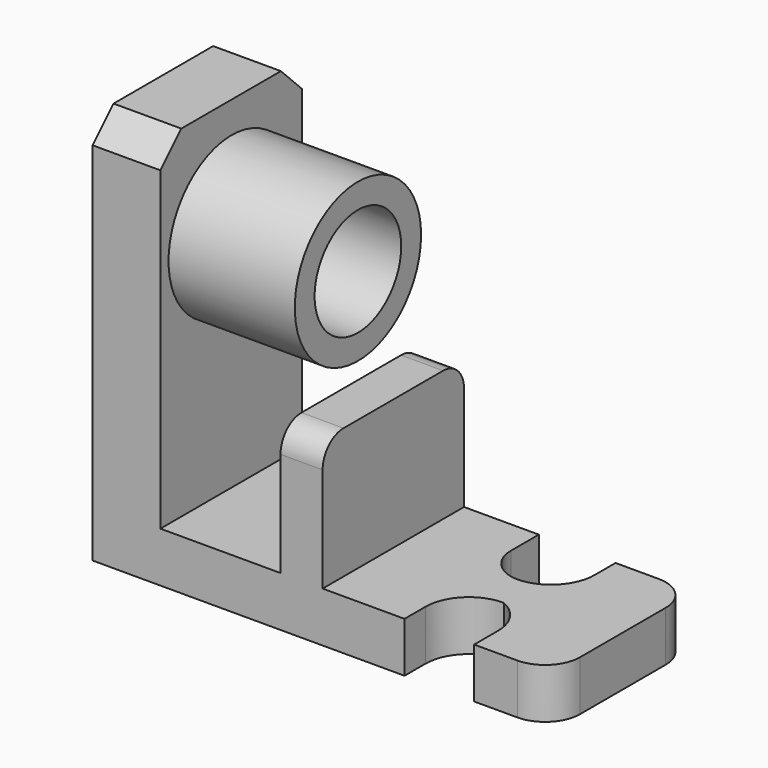
from build123d import *

# Parameters (mm, degrees)
F0_W         = 7.7837631106
F0_H         = 20.3025210649
F1_DEPTH     = 45
F2_SIZE      = 3
F4_W         = 20.3025210649
F4_H         = 5.7593202218
F5_DEPTH     = 45
F6_W         = 4.8367418349
F6_H         = 20.3025210649
F7_DEPTH     = 15
F8_R         = 3
F9_R         = 4
F10_W        = 8
F10_H        = 8
F11_DEPTH    = 25
F12_R        = 5
F13_T1_DEPTH = 5.7593202218
F15_DEPTH    = 25
F16_R        = 4
F17_T1_DEPTH = 5.7593202218
F3_R         = 9.0694207408
F3_R_2       = 6.2159496591
F18_DEPTH    = 14.5


# Not quite as in the source:
# - a fillet or chamfer that OpenCascade refuses, or shapes differently, is made with other operations: its cross-section is extruded or revolved along the edge and cut away or added


with BuildPart() as f1:
    # F0 (on Top) → F1 (new body)
    with BuildSketch(Plane.XY):
        with Locations((-49.9853566289, -10.1512605324)):
            Rectangle(F0_W, F0_H)
    extrude(amount=F1_DEPTH)

    # F2
    f2_edges = [f1.edges().sort_by_distance(p)[0] for p in [
        (-49.985357, -20.302521, 45),
        (-49.985357, 0, 45),
    ]]
    chamfer(f2_edges, length=F2_SIZE)

    # F4 (on face) → F5 (join)
    with BuildSketch(Plane.YZ.offset(-46.0934750736)):
        with Locations((-10.1512605324, 2.8796601109)):
            Rectangle(F4_W, F4_H)
    extrude(amount=F5_DEPTH)

    # F6 (on face) → F7 (join)
    with BuildSketch(Plane.XY.offset(5.7593202218)):
        with Locations((-29.8752058297, -10.1512605324)):
            Rectangle(F6_W, F6_H)
    extrude(amount=F7_DEPTH)

    # F8
    f8_edges = [f1.edges().sort_by_distance(p)[0] for p in [
        (-29.875206, 0, 20.75932),
        (-29.875206, -20.302521, 20.75932),
    ]]
    fillet(f8_edges, radius=F8_R)

    # F9
    f9_edges = [f1.edges().sort_by_distance(p)[0] for p in [
        (-1.093475, -20.302521, 2.87966),
        (-1.093475, 0, 2.87966),
    ]]
    fillet(f9_edges, radius=F9_R)

    # F10 (on face) → F11 (cut)
    with BuildSketch(Plane.XY.offset(5.7593202218)):
        with Locations((-14.0476680398, -16.3025210649)):
            Rectangle(F10_W, F10_H)
    extrude(amount=-F11_DEPTH, mode=Mode.SUBTRACT)

    # F12
    f12_edges = [f1.edges().sort_by_distance(p)[0] for p in [
        (-18.047668, -12.302521, 2.87966),
    ]]
    fillet(f12_edges, radius=F12_R)

    # F13: fillet of radius 5 on 1 edges, made by hand

    # F13_s2 → F13_t1 (join)
    with BuildSketch(Plane.XY):
        with BuildLine():
            ThreePointArc((-13.0476680398, -12.3025210649), (-10.8643679071, -14.1464839723), (-10.0476680398, -16.8850967598))
            Line((-10.0476680398, -16.8850967598), (-10.0476680398, -12.3025210649))
            Line((-10.0476680398, -12.3025210649), (-13.0476680398, -12.3025210649))
        make_face()
    extrude(amount=F13_T1_DEPTH)

    # F14 (on face) → F15 (cut)
    with BuildSketch(Plane.XY.offset(5.7593202218)):
        Polygon((-10.0476680398, 0), (-10.8643679071, 0), (-18.8643679071, 0), (-18.8643679071, -8), (-10.0476680398, -8), align=None)
    extrude(amount=-F15_DEPTH, mode=Mode.SUBTRACT)

    # F16
    f16_edges = [f1.edges().sort_by_distance(p)[0] for p in [
        (-18.864368, -8, 2.87966),
    ]]
    fillet(f16_edges, radius=F16_R)

    # F17: fillet of radius 5 on 1 edges, made by hand

    # F17_s2 → F17_t1 (join)
    with BuildSketch(Plane.XY):
        with BuildLine():
            ThreePointArc((-14.8643679071, -8), (-11.4479110575, -6.4734834519), (-10.0476680398, -3.0033610235))
            Line((-10.0476680398, -3.0033610235), (-9.9476680398, -3.0033610235))
            Line((-9.9476680398, -3.0033610235), (-9.9476680398, -8))
            Line((-9.9476680398, -8), (-10.0476680398, -8.1))
            ThreePointArc((-10.0476680398, -8.1), (-12.4560179735, -8.1), (-14.8607019045, -8.0999327795))
            Line((-14.8607019045, -8.0999327795), (-14.8643679071, -8))
        make_face()
    extrude(amount=F17_T1_DEPTH)

    # F3 (on face) → F18 (join)
    with BuildSketch(Plane.YZ.offset(-46.0934750736)):
        with Locations((-10.0637087598, 32.3379710317)):
            Circle(F3_R)
        with Locations((-10.0637087598, 32.3379710317)):
            Circle(F3_R_2, mode=Mode.SUBTRACT)
    extrude(amount=F18_DEPTH)


solid = f1.part
